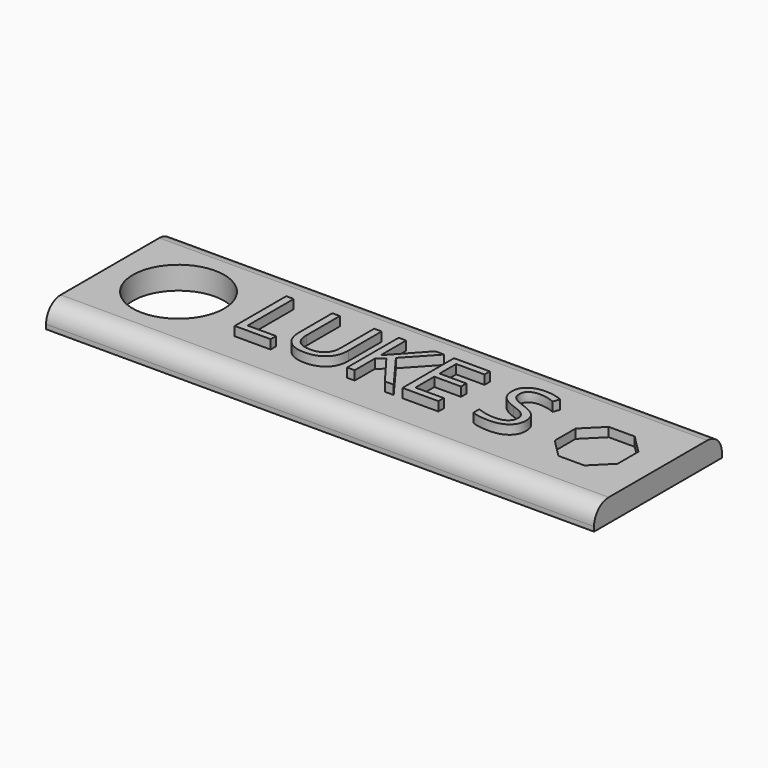
from build123d import *

# Parameters (mm, degrees)
F0_W         = 120
F0_H         = 35
F0_R         = 10
F1_DEPTH     = 5
F2_R         = 4
F3_R         = 4
F4_TEXT_SIZE = 19.7451419404
F6_DEPTH     = 2
F7_DEPTH     = 2


# Not quite as in the source:
# - Text() gives the source's letters only with a copy of the font that has no kerning and outlines rounded to 1/6400 em; it was checked with that copy


with BuildPart() as f1:
    # F0 (on Top) → F1 (new body)
    with BuildSketch(Plane.XY):
        Rectangle(F0_W, F0_H)
        with Locations((-45, 0)):
            Circle(F0_R, mode=Mode.SUBTRACT)
    extrude(amount=F1_DEPTH)

    # F2
    f2_edges = [f1.edges().sort_by_distance(p)[0] for p in [
        (0, -17.5, 5),
    ]]
    fillet(f2_edges, radius=F2_R)

    # F3
    f3_edges = [f1.edges().sort_by_distance(p)[0] for p in [
        (0, 17.5, 5),
    ]]
    fillet(f3_edges, radius=F3_R)

    # F4 (on face) → F6 (join)
    with BuildSketch(Plane.XY.offset(5)):
        with Locations((-29.1208922863, -6.8789552897)):
            Text('LUKE S', F4_TEXT_SIZE, font='Open Sans', text_align=(TextAlign.LEFT, TextAlign.BOTTOM))
    extrude(amount=F6_DEPTH)

    # F5 (on face) → F7 (cut)
    with BuildSketch(Plane.XY.offset(5)):
        Polygon((43.6978480659, -6.8789543584), (49.3965604463, -6.8789543584), (53.4261586145, -2.8493561902), (53.4261586145, 2.8493561902), (49.3965604463, 6.8789543584), (43.6978480659, 6.8789543584), (39.6682498977, 2.8493561902), (39.6682498977, -2.8493561902), align=None)
    extrude(amount=-F7_DEPTH, mode=Mode.SUBTRACT)


solid = f1.part
